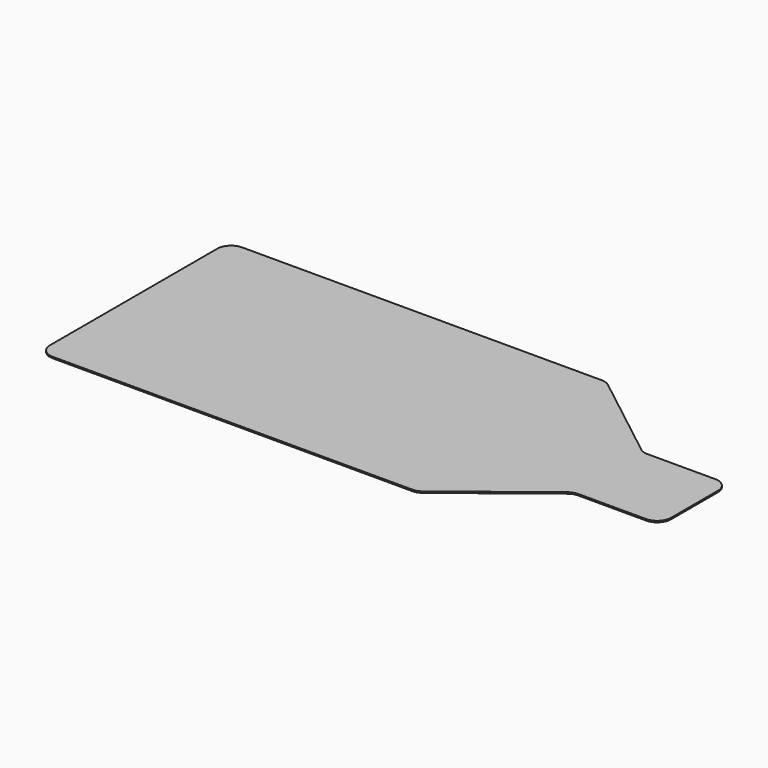
from build123d import *

# Parameters (mm, degrees)
F1_DEPTH = 0.127


# Not quite as in the source:
# - the program builds the solid bodies; features that only make, move or delete a surface that nothing else refers to are left out


with BuildPart() as f1:
    # F0 (on Top) → F1 (new body)
    with BuildSketch(Plane.XY):
        with BuildLine():
            Line((0, -2.6924), (0, 0))
            Line((0, 0), (0, 2.6924))
            ThreePointArc((0, 2.6924), (-0.3719743879, 3.5904256121), (-1.27, 3.9624))
            Line((-1.27, 3.9624), (-7.4879951317, 3.9624))
            ThreePointArc((-7.4879951317, 3.9624), (-7.9010514025, 4.0314484951), (-8.2691928483, 4.2310857998))
            Line((-8.2691928483, 4.2310857998), (-16.4196071517, 10.5898142002))
            ThreePointArc((-16.4196071517, 10.5898142002), (-16.7877485975, 10.7894515049), (-17.2008048683, 10.8585))
            Line((-17.2008048683, 10.8585), (-50.165, 10.8585))
            ThreePointArc((-50.165, 10.8585), (-51.0630256121, 10.4865256121), (-51.435, 9.5885))
            Line((-51.435, 9.5885), (-51.435, 0))
            Line((-51.435, 0), (-51.435, -9.5885))
            ThreePointArc((-51.435, -9.5885), (-51.0630256121, -10.4865256121), (-50.165, -10.8585))
            Line((-50.165, -10.8585), (-17.2008048683, -10.8585))
            ThreePointArc((-17.2008048683, -10.8585), (-16.7877485975, -10.7894515049), (-16.4196071517, -10.5898142002))
            Line((-16.4196071517, -10.5898142002), (-8.2691928483, -4.2310857998))
            ThreePointArc((-8.2691928483, -4.2310857998), (-7.9010514025, -4.0314484951), (-7.4879951317, -3.9624))
            Line((-7.4879951317, -3.9624), (-1.27, -3.9624))
            ThreePointArc((-1.27, -3.9624), (-0.3719743879, -3.5904256121), (0, -2.6924))
        make_face()
    extrude(amount=F1_DEPTH)


solid = f1.part
